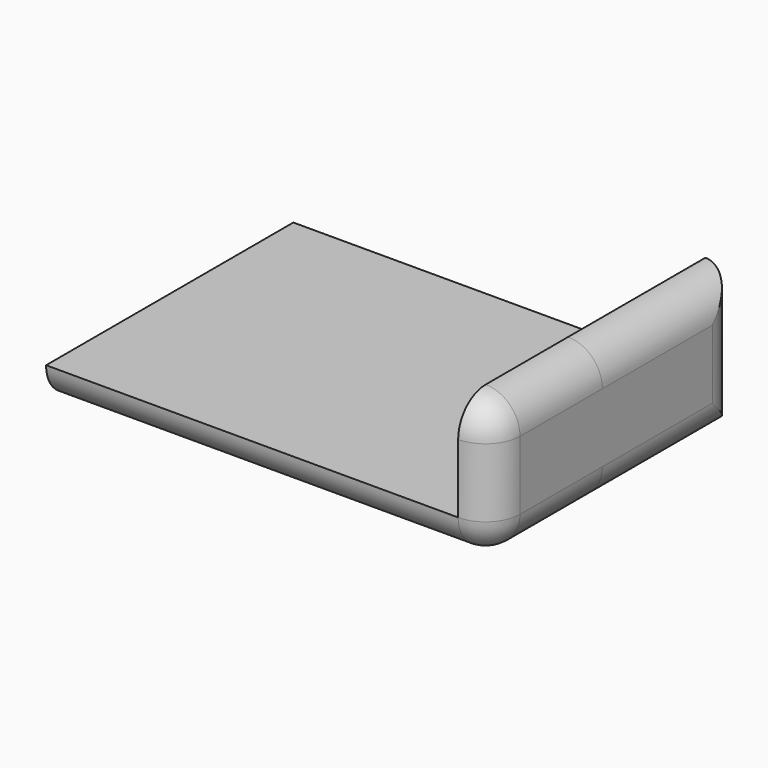
from build123d import *

# Parameters (mm, degrees)
F1_DEPTH = 45
F2_R     = 4.99999
F3_R     = 4.99999
F4_DEPTH = 25
F5_R     = 4.99999


# Not quite as in the source:
# - a fillet or chamfer is up to 0.001 mm smaller than in the source, because OpenCascade refuses the exact size


with BuildPart() as f1:
    # F0 (on Front) → F1 (new body)
    with BuildSketch(Plane.XZ):
        Polygon((0, 15), (0, 0), (-60, 0), (-60, -5), (5, -5), (5, 15), align=None)
    extrude(amount=F1_DEPTH)

    # F2 (radius 5 in the source; OpenCascade refuses exactly that, so slightly less here)
    f2_edges = [f1.edges().sort_by_distance(p)[0] for p in [
        (5, -22.5, 15),
    ]]
    fillet(f2_edges, radius=F2_R)

    # F3 (radius 5 in the source; OpenCascade refuses exactly that, so slightly less here)
    f3_edges = [f1.edges().sort_by_distance(p)[0] for p in [
        (5, -45, 2.500005),
        (-27.5, -45, -5),
        (3.535537, -45, 13.535537),
        (-27.5, 0, -5),
        (5, 0, 2.500005),
        (5, -22.5, -5),
    ]]
    fillet(f3_edges, radius=F3_R)

    # F0 (on Front) → F4 (join)
    with BuildSketch(Plane.XZ):
        Polygon((0, 15), (0, 0), (-60, 0), (-60, -5), (5, -5), (5, 15), align=None)
    extrude(amount=F4_DEPTH)

    # F5 (radius 5 in the source; OpenCascade refuses exactly that, so slightly less here)
    f5_edges = [f1.edges().sort_by_distance(p)[0] for p in [
        (5, -12.5, 15),
        (5, -12.5, -5),
        (5, 0, 5),
    ]]
    fillet(f5_edges, radius=F5_R)


solid = f1.part
